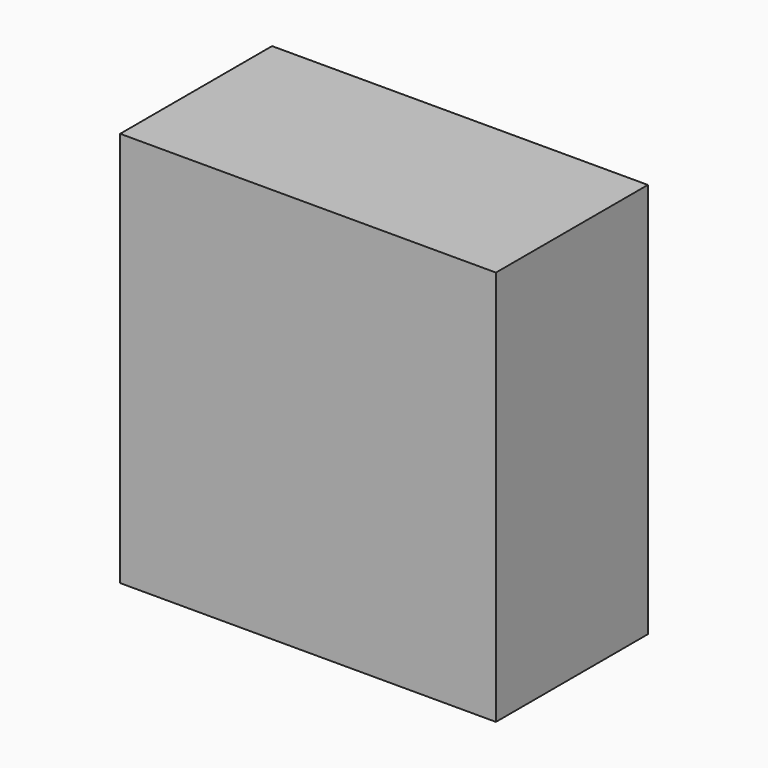
from build123d import *

# Parameters (mm, degrees)
F0_W     = 9.5
F0_H     = 4.8
F1_DEPTH = 10


# Not quite as in the source:
# - a feature names something its author has since deleted; it is built from what else it names


with BuildPart() as f1:
    # F0 (on Top) → F1 (new body)
    with BuildSketch(Plane.XY):
        with Locations((-4.75, 2.4)):
            Rectangle(F0_W, F0_H)
    extrude(amount=F1_DEPTH)


solid = f1.part
